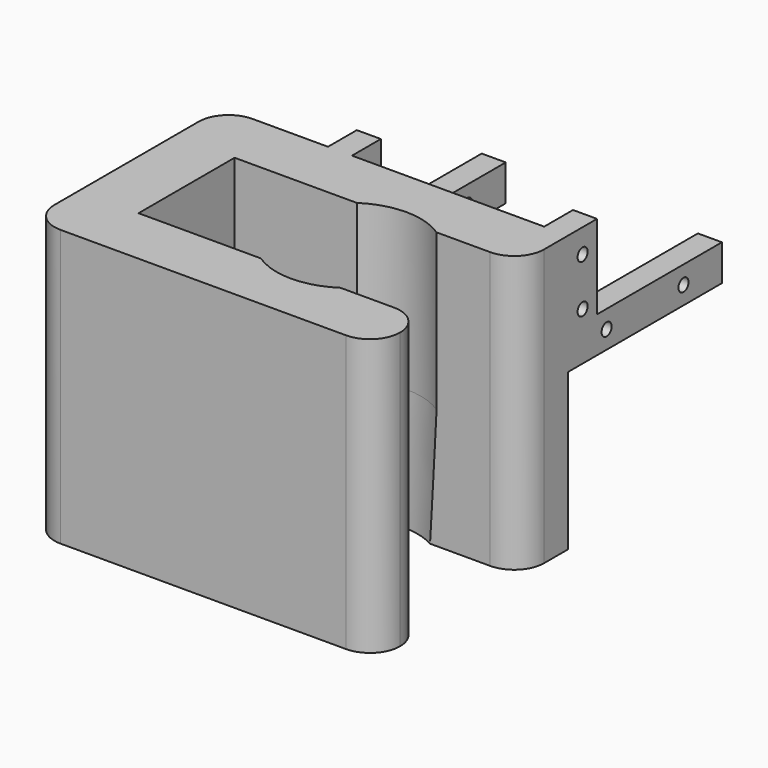
from build123d import *

# Parameters (mm, degrees)
F1_DEPTH        = 20
F2_DEPTH        = 26
F4_W            = 12
F4_H            = 26
F8_R            = 4.99999
F7_W            = 4
F7_H            = 20
F9_DEPTH        = 6
F10_W           = 4
F10_H           = 6
F11_DEPTH       = 26
F13_D           = 2.1
F14_R           = 11
F15_DEPTH       = 10
F16_D           = 2.1
F16_CBORE_D     = 3.5
F16_CBORE_DEPTH = 6
F18_D           = 2.1
F18_CBORE_D     = 3.7
F18_CBORE_DEPTH = 7


# Not quite as in the source:
# - a fillet or chamfer is up to 0.001 mm smaller than in the source, because OpenCascade refuses the exact size
# - a feature names something its author has since deleted; it is built from what else it names


with BuildPart() as f1:
    # F0 (on Top) → F1 (new body)
    with BuildSketch(Plane.XY):
        Polygon((30, 20), (-27.5520200282, 20), (-27.5520200282, -20), (30, -20), (30, -10), (-17.5520200282, -10), (-17.5520200282, 10), (30, 10), align=None)
    extrude(amount=-F1_DEPTH)

    # F0 (on Top) → F2 (join)
    with BuildSketch(Plane.XY):
        Polygon((30, 20), (-27.5520200282, 20), (-27.5520200282, -20), (30, -20), (30, -10), (-17.5520200282, -10), (-17.5520200282, 10), (30, 10), align=None)
    extrude(amount=F2_DEPTH)

    # F4 (on plane+point) → F5 (revolve, cut)
    with BuildSketch(Plane.YZ.offset(9.4479799718)):
        Polygon((12, 0), (0, 0), (0, -20), (11.4343625836, -20), align=None)
    revolve(axis=Axis((9.4479799718, 0, -10), (0, 0, -1)), mode=Mode.SUBTRACT)

    # F4 (on plane+point) → F6 (revolve, cut)
    with BuildSketch(Plane.YZ.offset(9.4479799718)):
        with Locations((6, 13)):
            Rectangle(F4_W, F4_H)
    revolve(axis=Axis((9.4479799718, 0, 13), (0, 0, 1)), mode=Mode.SUBTRACT)

    # F8 (radius 5 in the source; OpenCascade refuses exactly that, so slightly less here)
    f8_edges = [f1.edges().sort_by_distance(p)[0] for p in [
        (30, -10, 3),
        (30, 10, 3),
        (30, -20, 3),
        (-27.55202, -20, 3),
        (-27.55202, 20, 3),
    ]]
    fillet(f8_edges, radius=F8_R)

    # F7 (on face) → F9 (join)
    with BuildSketch(Plane(origin=(0, 20, 0), x_dir=(-1, 0, 0), z_dir=(0, 1, 0))):
        with Locations((-28, 16)):
            Rectangle(F7_W, F7_H)
        with Locations((8, 16)):
            Rectangle(F7_W, F7_H)
    extrude(amount=F9_DEPTH)

    # F10 (on face) → F11 (join)
    with BuildSketch(Plane(origin=(0, 26, 0), x_dir=(-1, 0, 0), z_dir=(0, 1, 0))):
        with Locations((-28, 9)):
            Rectangle(F10_W, F10_H)
        with Locations((8, 9)):
            Rectangle(F10_W, F10_H)
    extrude(amount=F11_DEPTH)

    # F13 (through all)
    with Locations(Plane.YZ.offset(30)):
        with Locations((23, 22), (23, 14), (28, 9), (44, 9)):
            Hole(F13_D / 2)

    # F18 (through all)
    with Locations(Plane.YZ.offset(-17.5520200282)):
        with Locations((-8, -1), (0, -1), (8, -1), (8, -9.0000019357), (8, -17), (0, -17), (-8, -17), (-8, -9.0000019357)):
            CounterBoreHole(F18_D / 2, F18_CBORE_D / 2, F18_CBORE_DEPTH)


with BuildPart() as f15:
    # F14 (on Front) → F15 (new body)
    with BuildSketch(Plane.XZ):
        Circle(F14_R)
    extrude(amount=-F15_DEPTH)

    # F16 (through all)
    with Locations(Plane.XZ):
        with Locations((0, 8), (8, 0), (0, -8), (-8, 0)):
            CounterBoreHole(F16_D / 2, F16_CBORE_D / 2, F16_CBORE_DEPTH)


solid = Compound([f1.part, f15.part])
